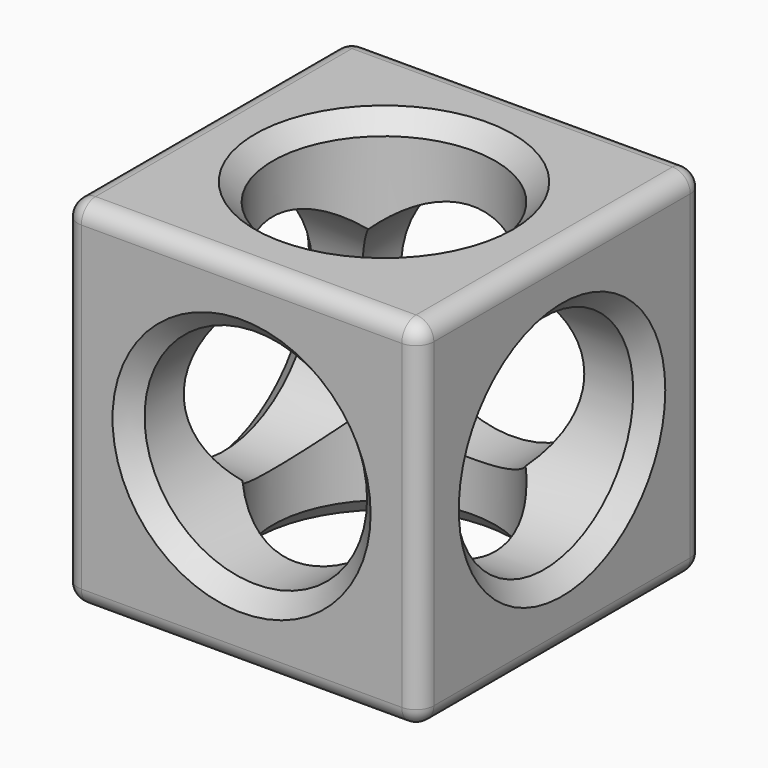
from build123d import *

# Parameters (mm, degrees)
F0_W         = 101.6
F0_H         = 101.6
F1_DEPTH     = 101.6
F2_R         = 31.75
F1_FACE1_W   = 101.6
F1_FACE1_H   = 101.6
F3_DEPTH     = 101.6
F4_R         = 31.75
F5_DEPTH     = 101.6
F6_R         = 31.75
F7_DEPTH     = 101.6
F8_R         = 5.08
F9_T1_DEPTH  = 91.44
F9_S5_W      = 5.08
F9_S5_H      = 5.08
F9_T6_DEPTH  = 5.08
F9_S11_W     = 5.08
F9_S11_H     = 5.08
F9_T12_DEPTH = 5.08
F10_SIZE     = 5.08


# Not quite as in the source:
# - a fillet or chamfer that OpenCascade refuses, or shapes differently, is made with other operations: its cross-section is extruded or revolved along the edge and cut away or added


with BuildPart() as f1:
    # F0 (on Top) → F1 (new body)
    with BuildSketch(Plane.XY):
        with Locations((50.8, 50.8)):
            Rectangle(F0_W, F0_H)
    extrude(amount=F1_DEPTH)

    # F2 (on face) + F1_face1 (on face) → F3 (cut)
    with BuildSketch(Plane.YZ.offset(101.6)):
        with Locations((50.8, 50.8)):
            Circle(F2_R)
    with BuildSketch(Plane(origin=(0, 50.8, 50.8), x_dir=(0, -1, 0), z_dir=(-1, 0, 0))):
        Rectangle(F1_FACE1_W, F1_FACE1_H)
    extrude(amount=-F3_DEPTH, dir=(1, 0, 0), mode=Mode.SUBTRACT)

    # F4 (on face) → F5 (cut)
    with BuildSketch(Plane.XZ):
        with Locations((50.8, 50.8)):
            Circle(F4_R)
    extrude(amount=-F5_DEPTH, mode=Mode.SUBTRACT)

    # F6 (on face) → F7 (cut)
    with BuildSketch(Plane(origin=(0, 0, 0), x_dir=(1, 0, 0), z_dir=(0, 0, -1))):
        with Locations((50.8, -50.8)):
            Circle(F6_R)
    extrude(amount=-F7_DEPTH, mode=Mode.SUBTRACT)

    # F8
    f8_edges = [f1.edges().sort_by_distance(p)[0] for p in [
        (50.8, 0, 101.6),
        (101.6, 50.8, 101.6),
        (50.8, 101.6, 101.6),
        (0, 50.8, 101.6),
        (101.6, 101.6, 50.8),
        (101.6, 0, 50.8),
        (101.6, 50.8, 0),
        (50.8, 101.6, 0),
        (0, 101.6, 50.8),
        (50.8, 0, 0),
        (0, 0, 50.8),
    ]]
    fillet(f8_edges, radius=F8_R)

    # F9: fillet of radius 5.08 on 1 edges, made by hand

    # F9_s2 → F9_t1 (cut)
    with BuildSketch(Plane.XZ.offset(-96.52)):
        with BuildLine():
            ThreePointArc((0, 5.08), (1.4878975516, 1.4878975516), (5.08, 0))
            Line((5.08, 0), (0, 0))
            Line((0, 0), (0, 5.08))
        make_face()
    extrude(amount=F9_T1_DEPTH, mode=Mode.SUBTRACT)


with BuildPart() as f9_tool4:
    # F9_s5 → F9_t6 (new body)
    with BuildSketch(Plane.YZ.offset(5.08)):
        with Locations((99.06, 2.54)):
            Rectangle(F9_S5_W, F9_S5_H)
    extrude(amount=-F9_T6_DEPTH)

    # F9_s7 → F9_t8 (revolve, cut)
    with BuildSketch(Plane(origin=(5.08, 96.52, 5.08), x_dir=(0, -0.7071067812, 0.7071067812), z_dir=(0, -0.7071067812, -0.7071067812))):
        with BuildLine():
            ThreePointArc((0, -5.08), (5.08, 0), (0, 5.08))
            Line((0, 5.08), (0, -5.08))
        make_face()
    revolve(axis=Axis((5.08, 96.52, 5.08), (-1, 0, 0)), mode=Mode.SUBTRACT)


with BuildPart() as f1_1:
    add(f1.part)

    # F9_t3: cut F9_tool4
    add(f9_tool4.part, mode=Mode.SUBTRACT)


with BuildPart() as f9_tool10:
    # F9_s11 → F9_t12 (new body)
    with BuildSketch(Plane.YZ.offset(5.08)):
        with Locations((2.54, 2.54)):
            Rectangle(F9_S11_W, F9_S11_H)
    extrude(amount=-F9_T12_DEPTH)

    # F9_s13 → F9_t14 (revolve, cut)
    with BuildSketch(Plane(origin=(5.08, 5.08, 5.08), x_dir=(0, 0.7071067812, 0.7071067812), z_dir=(0, -0.7071067812, 0.7071067812))):
        with BuildLine():
            ThreePointArc((0, -5.08), (5.08, 0), (0, 5.08))
            Line((0, 5.08), (0, -5.08))
        make_face()
    revolve(axis=Axis((5.08, 5.08, 5.08), (-1, 0, 0)), mode=Mode.SUBTRACT)


with BuildPart() as f1_2:
    add(f1_1.part)

    # F9_t9: cut F9_tool10
    add(f9_tool10.part, mode=Mode.SUBTRACT)

    # F10
    f10_edges = [f1_2.edges().sort_by_distance(p)[0] for p in [
        (101.6, 19.05, 50.8),
        (0, 19.05, 50.8),
        (19.05, 50.8, 0),
        (19.05, 0, 50.8),
        (19.05, 50.8, 101.6),
        (19.05, 101.6, 50.8),
    ]]
    chamfer(f10_edges, length=F10_SIZE)


solid = f1_2.part
